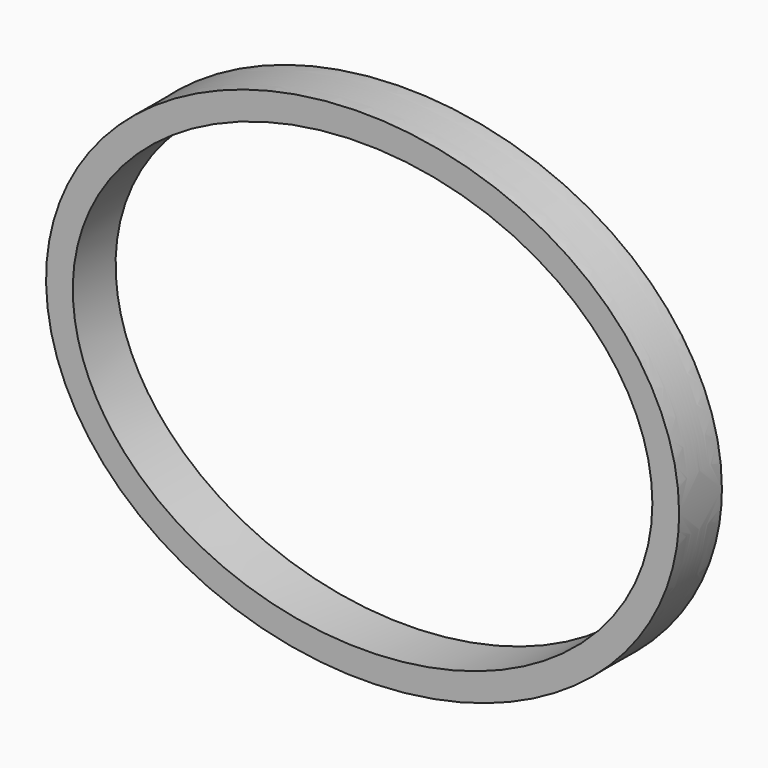
from build123d import *

# Parameters (mm, degrees)
F1_DEPTH = 6


# Not quite as in the source:
# - the dataset's text gives a spline's control points without its knots; the knots are read off the source's solid


with BuildPart() as f1:
    # F0 (on Front) → F1 (new body)
    with BuildSketch(Plane.XZ):
        with BuildLine():
            add(Edge.make_bspline(
                [(35.5, 0), (35.5, 0.4782664444), (35.4690728995, 1.4347993331), (35.2853198307, 3.3313716528), (34.830857782, 5.6680854172), (33.940087853, 8.3907113774), (32.7196850061, 11.0099347498), (31.1856661913, 13.5059353476), (29.3536926796, 15.8611484476), (27.5906148879, 17.6934458109), (26.0458457556, 19.0729617457), (24.8197773382, 20.0641032105), (23.5356609184, 21.0038743942), (21.7607020267, 22.1797537651), (19.4268792103, 23.5076242103), (16.4664284421, 24.8692312016), (13.3674951304, 25.9953656663), (10.1512797187, 26.8813999683), (6.8386442643, 27.5221713908), (4.0144383029, 27.846914894), (1.7282069584, 27.9779633024), (0, 28.0110183488), (-1.7282069584, 27.9779633024), (-4.0144383029, 27.846914894), (-6.8386442643, 27.5221713908), (-10.1512797187, 26.8813999683), (-13.3674951304, 25.9953656663), (-16.4664284421, 24.8692312016), (-19.4268792103, 23.5076242103), (-21.7607020267, 22.1797537651), (-23.5356609184, 21.0038743942), (-24.8197773382, 20.0641032105), (-26.0458457556, 19.0729617457), (-27.5906148879, 17.6934458109), (-29.3536926796, 15.8611484476), (-31.1856661913, 13.5059353476), (-32.7196850061, 11.0099347498), (-33.940087853, 8.3907113774), (-34.830857782, 5.6680854172), (-35.2853198307, 3.3313716528), (-35.4690728995, 1.4347993331), (-35.5154635503, 0), (-35.4690728995, -1.4347993331), (-35.2853198307, -3.3313716528), (-34.830857782, -5.6680854172), (-33.940087853, -8.3907113774), (-32.7196850061, -11.0099347498), (-31.1856661913, -13.5059353476), (-29.3536926796, -15.8611484476), (-27.5906148879, -17.6934458109), (-26.0458457556, -19.0729617457), (-24.8197773382, -20.0641032105), (-23.5356609184, -21.0038743942), (-21.7607020267, -22.1797537651), (-19.4268792103, -23.5076242103), (-16.4664284421, -24.8692312016), (-13.3674951304, -25.9953656663), (-10.1512797187, -26.8813999683), (-6.8386442643, -27.5221713908), (-4.0144383029, -27.846914894), (-1.7282069584, -27.9779633024), (0, -28.0110183488), (1.7282069584, -27.9779633024), (4.0144383029, -27.846914894), (6.8386442643, -27.5221713908), (10.1512797187, -26.8813999683), (13.3674951304, -25.9953656663), (16.4664284421, -24.8692312016), (19.4268792103, -23.5076242103), (21.7607020267, -22.1797537651), (23.5356609184, -21.0038743942), (24.8197773382, -20.0641032105), (26.0458457556, -19.0729617457), (27.5906148879, -17.6934458109), (29.3536926796, -15.8611484476), (31.1856661913, -13.5059353476), (32.7196850061, -11.0099347498), (33.940087853, -8.3907113774), (34.830857782, -5.6680854172), (35.2853198307, -3.3313716528), (35.4690728995, -1.4347993331), (35.5, -0.4782664444), (35.5, 0)],
                knots=[0, 0, 0, 0, 0.0078125, 0.015625, 0.03125, 0.046875, 0.0625, 0.078125, 0.09375, 0.109375, 0.1171875, 0.125, 0.1328125, 0.140625, 0.15625, 0.171875, 0.1875, 0.203125, 0.21875, 0.234375, 0.2421875, 0.25, 0.2578125, 0.265625, 0.28125, 0.296875, 0.3125, 0.328125, 0.34375, 0.359375, 0.3671875, 0.375, 0.3828125, 0.390625, 0.40625, 0.421875, 0.4375, 0.453125, 0.46875, 0.484375, 0.4921875, 0.5, 0.5078125, 0.515625, 0.53125, 0.546875, 0.5625, 0.578125, 0.59375, 0.609375, 0.6171875, 0.625, 0.6328125, 0.640625, 0.65625, 0.671875, 0.6875, 0.703125, 0.71875, 0.734375, 0.7421875, 0.75, 0.7578125, 0.765625, 0.78125, 0.796875, 0.8125, 0.828125, 0.84375, 0.859375, 0.8671875, 0.875, 0.8828125, 0.890625, 0.90625, 0.921875, 0.9375, 0.953125, 0.96875, 0.984375, 0.9921875, 1, 1, 1, 1], degree=3))
        make_face()
        with BuildLine():
            add(Edge.make_bspline(
                [(32.5, 0), (32.5, 43.3012701892), (-16.25, 21.6506350946), (-65, 0), (-16.25, -21.6506350946), (32.5, -43.3012701892), (32.5, 0)],
                knots=[0, 0, 0, 2.0943951024, 2.0943951024, 4.1887902048, 4.1887902048, 6.2831853072, 6.2831853072, 6.2831853072], degree=2, weights=[1, 0.5, 1, 0.5, 1, 0.5, 1]))
        make_face(mode=Mode.SUBTRACT)
    extrude(amount=F1_DEPTH)


solid = f1.part
